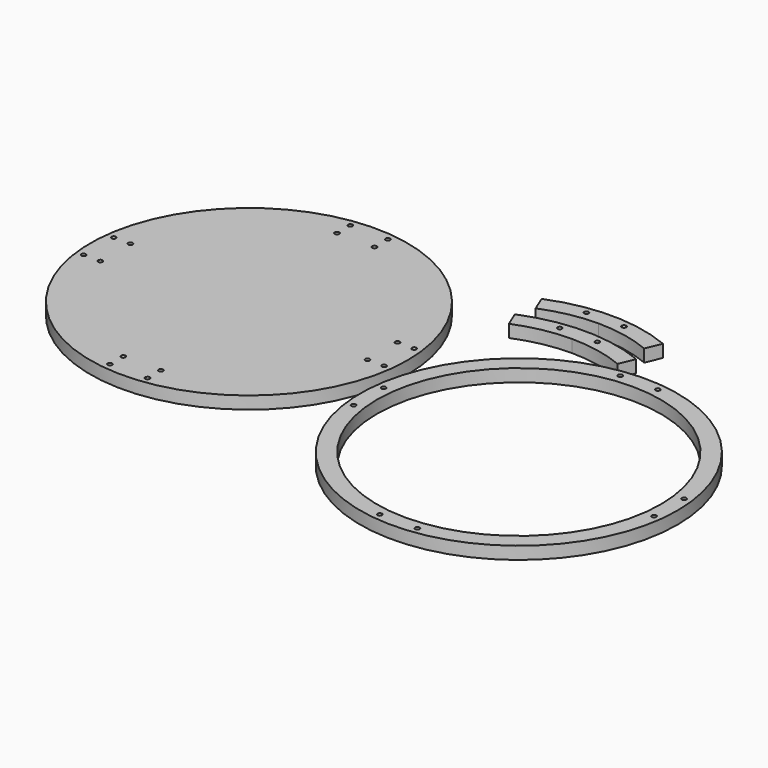
from build123d import *

# Parameters (mm, degrees)
F0_R     = 241.3
F0_R_2   = 3.429
F1_DEPTH = 19.05
F0_R_3   = 215.9


# Not quite as in the source:
# - a feature names something its author has since deleted; it is built from what else it names


with BuildPart() as f1:
    # F0 (on Top) → F1 (new body)
    with BuildSketch(Plane.XY):
        with Locations((-491.9811487198, 101.6)):
            Circle(F0_R)
        with Locations((-520.5561487198, -127)):
            Circle(F0_R_2, mode=Mode.SUBTRACT)
        with Locations((-520.5561487198, -101.6)):
            Circle(F0_R_2, mode=Mode.SUBTRACT)
        with Locations((-463.4061487198, -127)):
            Circle(F0_R_2, mode=Mode.SUBTRACT)
        with Locations((-463.4061487198, -101.6)):
            Circle(F0_R_2, mode=Mode.SUBTRACT)
        with Locations((-720.5811487198, 73.025)):
            Circle(F0_R_2, mode=Mode.SUBTRACT)
        with Locations((-695.1811487198, 73.025)):
            Circle(F0_R_2, mode=Mode.SUBTRACT)
        with Locations((-720.5811487198, 130.175)):
            Circle(F0_R_2, mode=Mode.SUBTRACT)
        with Locations((-695.1811487198, 130.175)):
            Circle(F0_R_2, mode=Mode.SUBTRACT)
        with Locations((-288.7811487198, 73.025)):
            Circle(F0_R_2, mode=Mode.SUBTRACT)
        with Locations((-263.3811487198, 73.025)):
            Circle(F0_R_2, mode=Mode.SUBTRACT)
        with Locations((-288.7811487198, 130.175)):
            Circle(F0_R_2, mode=Mode.SUBTRACT)
        with Locations((-263.3811487198, 130.175)):
            Circle(F0_R_2, mode=Mode.SUBTRACT)
        with Locations((-520.5561487198, 304.8)):
            Circle(F0_R_2, mode=Mode.SUBTRACT)
        with Locations((-520.5561487198, 330.2)):
            Circle(F0_R_2, mode=Mode.SUBTRACT)
        with Locations((-463.4061487198, 304.8)):
            Circle(F0_R_2, mode=Mode.SUBTRACT)
        with Locations((-463.4061487198, 330.2)):
            Circle(F0_R_2, mode=Mode.SUBTRACT)
    extrude(amount=F1_DEPTH)


with BuildPart() as f1b:
    # F0 (on Top) → F1, piece 2 (new body)
    with BuildSketch(Plane.XY):
        with BuildLine():
            ThreePointArc((-132.7304871559, 342.9), (-179.8057818584, 338.2634881613), (-225.0719993856, 324.532131195))
            Line((-225.0719993856, 324.532131195), (-215.3518402035, 301.0655910692))
            ThreePointArc((-215.3518402035, 301.0655910692), (-174.8504876792, 313.3515420391), (-132.7304871559, 317.5))
            ThreePointArc((-132.7304871559, 317.5), (-90.6104866326, 313.3515420391), (-50.1091341083, 301.0655910692))
            Line((-50.1091341083, 301.0655910692), (-40.3889749262, 324.532131195))
            ThreePointArc((-40.3889749262, 324.532131195), (-85.6551924534, 338.2634881613), (-132.7304871559, 342.9))
        make_face()
        with Locations((-161.3054871559, 330.2)):
            Circle(F0_R_2, mode=Mode.SUBTRACT)
        with Locations((-104.1554871559, 330.2)):
            Circle(F0_R_2, mode=Mode.SUBTRACT)
    extrude(amount=F1_DEPTH)


with BuildPart() as f1c:
    # F0 (on Top) → F1, piece 3 (new body)
    with BuildSketch(Plane.XY):
        with BuildLine():
            ThreePointArc((-132.7304871559, 292.1), (-179.8057818584, 287.4634881613), (-225.0719993856, 273.732131195))
            Line((-225.0719993856, 273.732131195), (-215.3518402035, 250.2655910692))
            ThreePointArc((-215.3518402035, 250.2655910692), (-174.8504876792, 262.5515420391), (-132.7304871559, 266.7))
            ThreePointArc((-132.7304871559, 266.7), (-90.6104866326, 262.5515420391), (-50.1091341083, 250.2655910692))
            Line((-50.1091341083, 250.2655910692), (-40.3889749262, 273.732131195))
            ThreePointArc((-40.3889749262, 273.732131195), (-85.6551924534, 287.4634881613), (-132.7304871559, 292.1))
        make_face()
        with Locations((-161.3054871559, 279.4)):
            Circle(F0_R_2, mode=Mode.SUBTRACT)
        with Locations((-104.1554871559, 279.4)):
            Circle(F0_R_2, mode=Mode.SUBTRACT)
    extrude(amount=F1_DEPTH)


with BuildPart() as f1d:
    # F0 (on Top) → F1, piece 4 (new body)
    with BuildSketch(Plane.XY):
        Circle(F0_R)
        with Locations((-28.575, -228.6)):
            Circle(F0_R_2, mode=Mode.SUBTRACT)
        with Locations((28.575, -228.6)):
            Circle(F0_R_2, mode=Mode.SUBTRACT)
        with Locations((-228.6, -28.575)):
            Circle(F0_R_2, mode=Mode.SUBTRACT)
        with Locations((-228.6, 28.575)):
            Circle(F0_R_2, mode=Mode.SUBTRACT)
        with Locations((228.6, -28.575)):
            Circle(F0_R_2, mode=Mode.SUBTRACT)
        Circle(F0_R_3, mode=Mode.SUBTRACT)
        with Locations((228.6, 28.575)):
            Circle(F0_R_2, mode=Mode.SUBTRACT)
        with Locations((-28.575, 228.6)):
            Circle(F0_R_2, mode=Mode.SUBTRACT)
        with Locations((28.575, 228.6)):
            Circle(F0_R_2, mode=Mode.SUBTRACT)
    extrude(amount=F1_DEPTH)


solid = Compound([f1.part, f1b.part, f1c.part, f1d.part])
